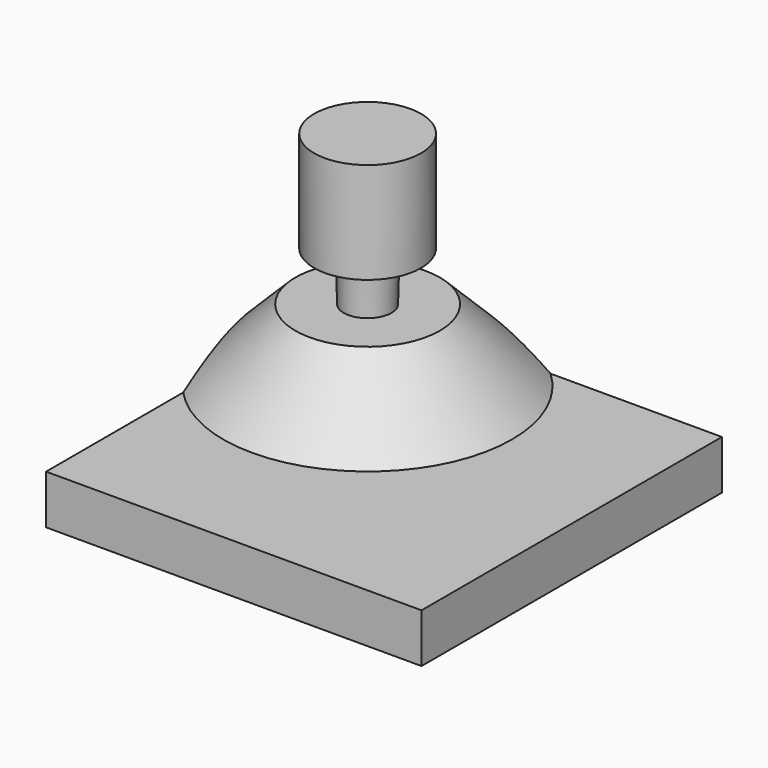
from build123d import *

# Parameters (mm, degrees)
F0_W          = 16.51
F0_H          = 16.51
F1_DEPTH      = 2.159
F2_R          = 3.175
F3_DEPTH      = 3.175
F3_DEPTH_BACK = 1.27
F4_R          = 1.04775
F5_DEPTH      = 5.08
F5_TAPER      = -1.5
F8_R          = 2.3495
F9_DEPTH      = 1.27
F10_R         = 2.3495
F10_R_2       = 1.3335
F11_DEPTH     = 3.175


# Not quite as in the source:
# - a fillet or chamfer that OpenCascade refuses, or shapes differently, is made with other operations: its cross-section is extruded or revolved along the edge and cut away or added


with BuildPart() as f1:
    # F0 (on Top) → F1 (new body)
    with BuildSketch(Plane.XY):
        Rectangle(F0_W, F0_H)
    extrude(amount=F1_DEPTH)

    # F2 (on face) → F3 (join, two sides)
    with BuildSketch(Plane.XY.offset(2.159)) as f3_sk:
        with Locations((-3.605306847, 3.605306847)):
            Circle(F2_R)
    extrude(amount=F3_DEPTH)
    extrude(f3_sk.sketch, amount=-F3_DEPTH_BACK)

    # F4 (on face) → F5 (join)
    with BuildSketch(Plane.XY.offset(5.334)):
        with Locations((-3.605306847, 3.605306847)):
            Circle(F4_R)
    extrude(amount=F5_DEPTH, taper=F5_TAPER)

    # F12: chamfer of 3.175 on 1 edges, made by hand


with BuildPart() as f9:
    # F8 (on offset) → F9 (new body)
    with BuildSketch(Plane.XY.offset(10.668)):
        with Locations((-3.605306847, 3.605306847)):
            Circle(F8_R)
    extrude(amount=F9_DEPTH)

    # F10 (on face) → F11 (join)
    with BuildSketch(Plane(origin=(0, 0, 10.668), x_dir=(1, 0, 0), z_dir=(0, 0, -1))):
        with Locations((-3.605306847, -3.605306847)):
            Circle(F10_R)
        with Locations((-3.605306847, -3.605306847)):
            Circle(F10_R_2, mode=Mode.SUBTRACT)
    extrude(amount=F11_DEPTH)


with BuildPart() as f12_tool2:
    # F12_s3 → F12_t4 (revolve)
    with BuildSketch(Plane.XZ.offset(-3.605306847)):
        Polygon((2.744693153, 2.159), (-0.430306847, 5.334), (-0.430306847, 2.159), align=None)
    revolve(axis=Axis((-3.605306847, 3.605306847, 2.159), (0, 0, 1)))

    split(bisect_by=Plane.XZ.offset(-8.255), keep=Keep.TOP)

    split(bisect_by=Plane.YZ.offset(-8.255), keep=Keep.TOP)

    split(bisect_by=Plane.XY.offset(5.334), keep=Keep.BOTTOM)


with BuildPart() as f1_1:
    add(f1.part)

    # F12_t1: union F12_tool2
    add(f12_tool2.part)


solid = Compound([f9.part, f1_1.part])
